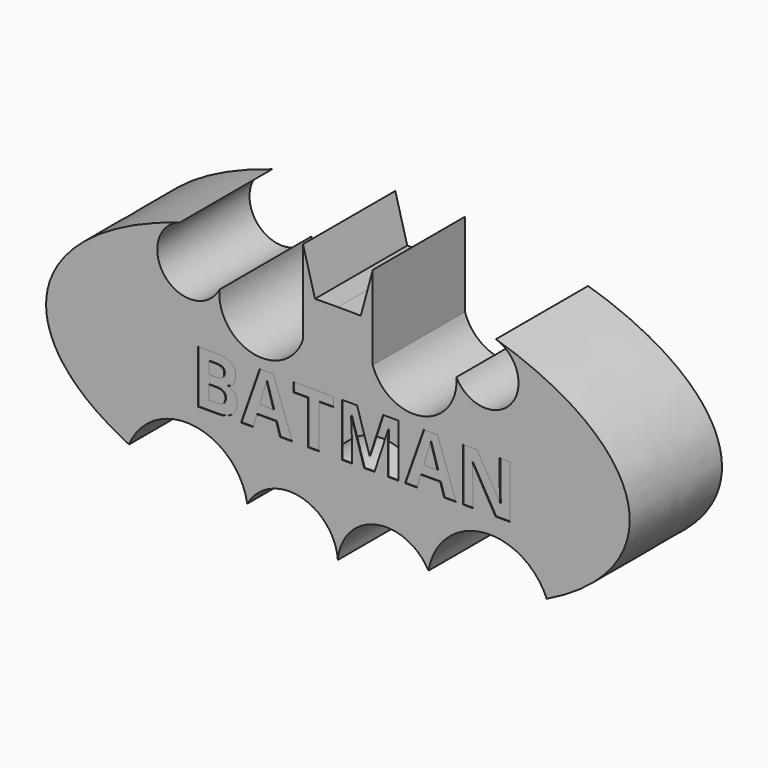
from build123d import *

# Parameters (mm, degrees)
F1_DEPTH     = 30
F2_TEXT_SIZE = 19.2911545229
F3_DEPTH     = 0.2


# Not quite as in the source:
# - Text() gives the source's letters only with a copy of the font that has no kerning and outlines rounded to 1/6400 em; it was checked with that copy


with BuildPart() as f1:
    # F0 (on Front) → F1 (new body)
    with BuildSketch(Plane.XZ):
        with BuildLine():
            ThreePointArc((-30.828340973, 18.0845544578), (-44.9441491849, 16.4436336767), (-41.093175472, 30.1227661034))
            add(Edge.make_bspline(
                [(-41.093175472, 30.1227661034), (-119.2258602368, 6.3751990886), (-54.3275669252, -25.0204650694)],
                knots=[2.1428841375, 2.1428841375, 2.1428841375, 3.9146955172, 3.9146955172, 3.9146955172], degree=2, weights=[1, 0.6325883149, 1]))
            ThreePointArc((-54.3275669252, -25.0204650694), (-37.609113326, -15.2234645359), (-23.5748211455, -28.5848474433))
            ThreePointArc((-23.5748211455, -28.5848474433), (-9.8609560996, -22.482189722), (0, -33.7991712348))
            ThreePointArc((0, -33.7991712348), (9.8609560996, -22.482189722), (23.5748211455, -28.5848474433))
            ThreePointArc((23.5748211455, -28.5848474433), (37.609113326, -15.2234645359), (54.3275669252, -25.0204650694))
            add(Edge.make_bspline(
                [(54.3275669252, -25.0204650694), (119.2258602368, 6.3751990886), (41.093175472, 30.1227661034)],
                knots=[5.5100824436, 5.5100824436, 5.5100824436, 7.2818938232, 7.2818938232, 7.2818938232], degree=2, weights=[1, 0.6325883149, 1]))
            ThreePointArc((41.093175472, 30.1227661034), (44.9441491849, 16.4436336767), (30.828340973, 18.0845544578))
            ThreePointArc((30.828340973, 18.0845544578), (21.8673086268, 6.2365758172), (9.0660702204, 13.7733519077))
            Line((9.0660702204, 13.7733519077), (9.0660702204, 35.5710034911))
            Line((9.0660702204, 35.5710034911), (5.9553950305, 24.0686364381))
            Line((5.9553950305, 24.0686364381), (0, 24.1161175072))
            Line((0, 24.1161175072), (-5.9553950305, 24.0686364381))
            Line((-5.9553950305, 24.0686364381), (-9.0660702204, 35.5710034911))
            Line((-9.0660702204, 35.5710034911), (-9.0660702204, 13.7733519077))
            ThreePointArc((-9.0660702204, 13.7733519077), (-21.8673086268, 6.2365758172), (-30.828340973, 18.0845544578))
        make_face()
    extrude(amount=F1_DEPTH)

    # F2 (on face) → F3 (cut)
    with BuildSketch(Plane.XZ.offset(30)):
        with Locations((-38.1690710783, -10.5314161628)):
            Text('BATMAN', F2_TEXT_SIZE, font='Open Sans', font_style=FontStyle.BOLD, text_align=(TextAlign.LEFT, TextAlign.BOTTOM))
    extrude(amount=-F3_DEPTH, mode=Mode.SUBTRACT)


solid = f1.part
